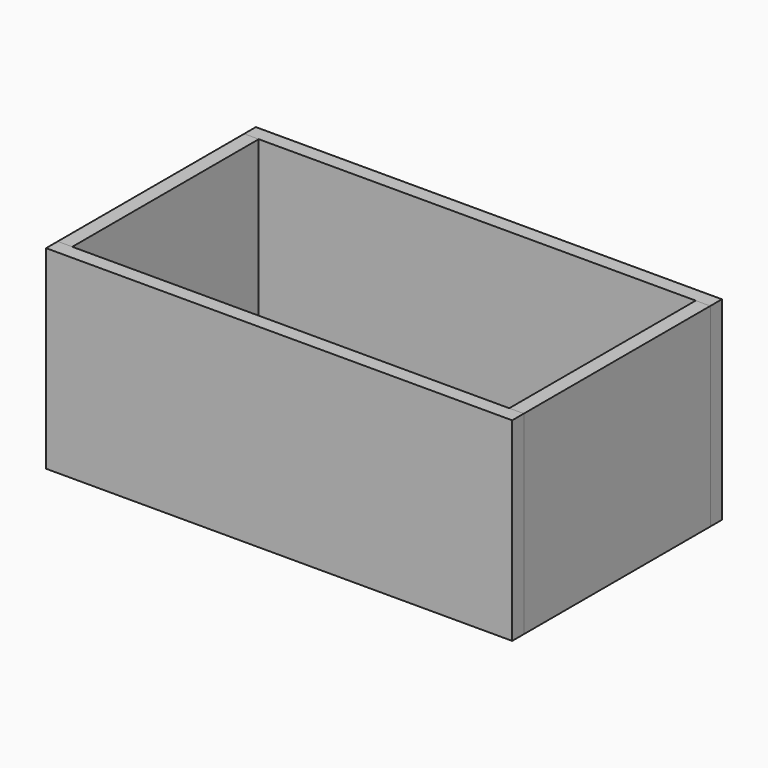
from build123d import *

# Parameters (mm, degrees)
F2_W     = 571.5
F2_H     = 304.8
F3_DEPTH = 19.05
F2_W_2   = 19.05
F4_DEPTH = 254
F5_DEPTH = 254


# Not quite as in the source:
# - a variable given as a bare number and used for a length is read in inches; the dataset says mm whatever the document's units were


with BuildPart() as f3:
    # F2 (on Top) → F3 (new body)
    with BuildSketch(Plane.XY):
        Rectangle(F2_W, F2_H)
    extrude(amount=F3_DEPTH)


with BuildPart() as f4:
    # F2 (on Top) → F4 (new body)
    with BuildSketch(Plane.XY):
        with Locations((-295.275, 0)):
            Rectangle(F2_W_2, F2_H)
    extrude(amount=F4_DEPTH)


with BuildPart() as f4b:
    # F2 (on Top) → F4, piece 2 (new body)
    with BuildSketch(Plane.XY):
        with Locations((295.275, 0)):
            Rectangle(F2_W_2, F2_H)
    extrude(amount=F4_DEPTH)


with BuildPart() as f5:
    # F2 (on Top) → F5 (new body)
    with BuildSketch(Plane.XY):
        Polygon((304.8, -152.4), (285.75, -152.4), (-285.75, -152.4), (-304.8, -152.4), (-304.8, -171.45), (304.8, -171.45), align=None)
    extrude(amount=F5_DEPTH)


with BuildPart() as f5b:
    # F2 (on Top) → F5, piece 2 (new body)
    with BuildSketch(Plane.XY):
        Polygon((-285.75, 152.4), (285.75, 152.4), (304.8, 152.4), (304.8, 171.45), (-304.8, 171.45), (-304.8, 152.4), align=None)
    extrude(amount=F5_DEPTH)


solid = Compound([f3.part, f4.part, f4b.part, f5.part, f5b.part])
